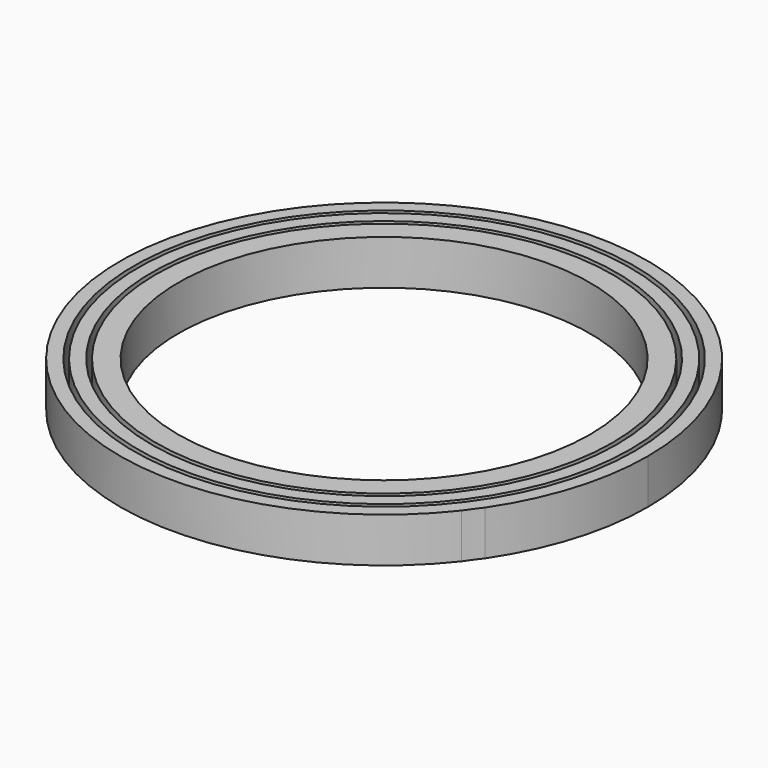
from build123d import *

# Parameters (mm, degrees)
F0_R     = 28
F1_DEPTH = 5
F0_R_2   = 25.5
F0_R_3   = 23
F0_R_4   = 27.5
F0_R_5   = 26


# Not quite as in the source:
# - a feature names something its author has since deleted; it is built from what else it names


with BuildPart() as f1:
    # F0 (on Top) → F1 (new body)
    with BuildSketch(Plane.XY):
        with BuildLine():
            ThreePointArc((24.4593593513, 43.5078885487), (28.211709456, 51.377387312), (29.5, 60))
            ThreePointArc((29.5, 60), (-8.622612688, 88.211709456), (-24.4593593513, 43.5078885487))
            ThreePointArc((-24.4593593513, 43.5078885487), (-23.8253683168, 42.6704704408), (-23.2239332129, 41.8093725747))
            ThreePointArc((-23.2239332129, 41.8093725747), (0, 30.5), (23.2239332129, 41.8093725747))
            ThreePointArc((23.2239332129, 41.8093725747), (23.8253683168, 42.6704704408), (24.4593593513, 43.5078885487))
        make_face()
        with Locations((0, 60)):
            Circle(F0_R, mode=Mode.SUBTRACT)
    extrude(amount=F1_DEPTH)


with BuildPart() as f1b:
    # F0 (on Top) → F1, piece 2 (new body)
    with BuildSketch(Plane.XY):
        with Locations((0, 60)):
            Circle(F0_R_2)
        with Locations((0, 60)):
            Circle(F0_R_3, mode=Mode.SUBTRACT)
    extrude(amount=F1_DEPTH)


with BuildPart() as f1c:
    # F0 (on Top) → F1, piece 3 (new body)
    with BuildSketch(Plane.XY):
        with Locations((0, 60)):
            Circle(F0_R_4)
        with Locations((0, 60)):
            Circle(F0_R_5, mode=Mode.SUBTRACT)
    extrude(amount=F1_DEPTH)


solid = Compound([f1.part, f1b.part, f1c.part])
